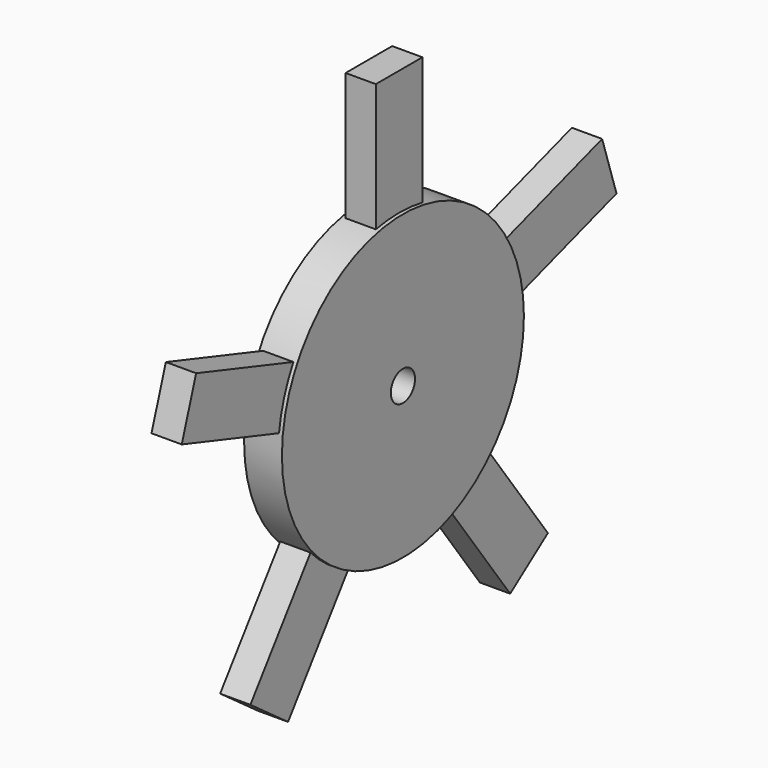
from build123d import *

# Parameters (mm, degrees)
F2_R     = 25.4
F2_R_2   = 2.54
F3_DEPTH = 3.175
F4_W     = 9.7803566605
F4_H     = 21.473386322
F5_DEPTH = 2.54


# Not quite as in the source:
# - the program builds the solid bodies; features that only make, move or delete a surface that nothing else refers to are left out


with BuildPart() as f3:
    # F2 (on Right) → F3 (new body, symmetric)
    with BuildSketch(Plane.YZ):
        Circle(F2_R)
        Circle(F2_R_2, mode=Mode.SUBTRACT)
    extrude(amount=F3_DEPTH, both=True)

    # F4 (on Right) → F5 (join, symmetric)
    with BuildSketch(Plane.YZ):
        with Locations((0, 35.6615032084)):
            Rectangle(F4_W, F4_H)
        Polygon((-45.638455211, 9.6869952197), (-25.2160512226, 3.0513539194), (-22.1937548034, 12.353025853), (-42.6161587919, 18.9886671533), align=None)
        Polygon((-23.3159381842, -40.4113040748), (-10.6941983874, -23.0389696135), (-18.6066731367, -17.2902202063), (-31.2284129336, -34.6625546676), align=None)
        Polygon((31.2284129336, -34.6625546676), (18.6066731367, -17.2902202063), (10.6941983874, -23.0389696135), (23.3159381842, -40.4113040748), align=None)
        Polygon((42.6161587919, 18.9886671533), (22.1937548034, 12.353025853), (25.2160512226, 3.0513539194), (45.638455211, 9.6869952197), align=None)
    extrude(amount=F5_DEPTH, both=True)


solid = f3.part
